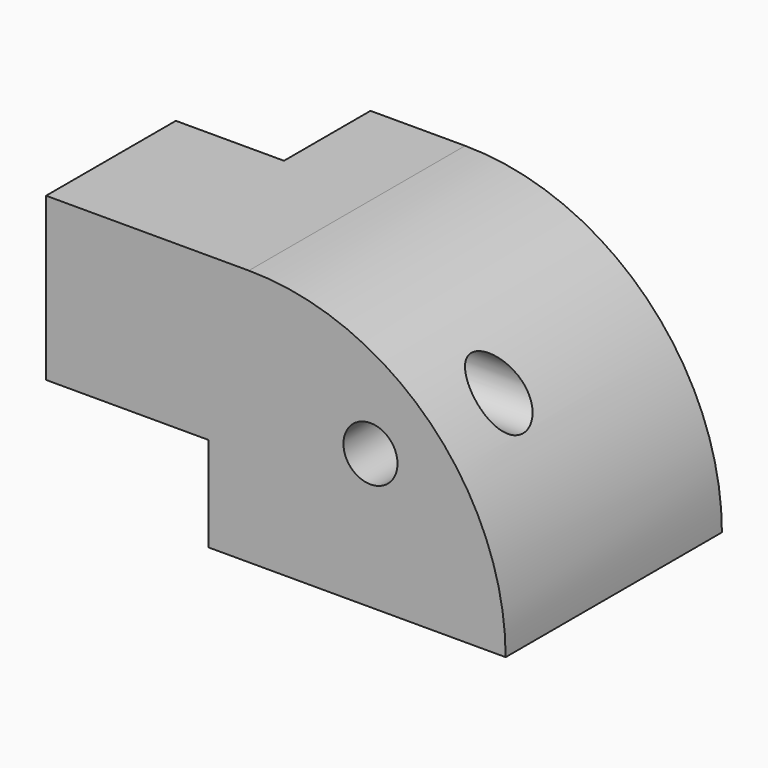
from build123d import *

# Parameters (mm, degrees)
F0_W      = 127
F0_H      = 120.65
F1_DEPTH  = 215.9
F2_W      = 76.2
F2_H      = 44.45
F3_DEPTH  = 127
F4_W      = 50.8
F4_H      = 76.2
F5_DEPTH  = 50.8
F8_D      = 25.4
F8_DEPTH  = 127
F8_TIP    = 7.6309298617
F9_R      = 120.64999
F10_DEPTH = 50.8
F13_D     = 25.4


# Not quite as in the source:
# - a fillet or chamfer is up to 0.001 mm smaller than in the source, because OpenCascade refuses the exact size
# - a feature of the source that left no trace in its solid (it failed there, or was rolled back) is left out


with BuildPart() as f1:
    # F0 (on Right) → F1 (new body)
    with BuildSketch(Plane.YZ):
        Rectangle(F0_W, F0_H)
    extrude(amount=F1_DEPTH)

    # F2 (on face) → F3 (cut)
    with BuildSketch(Plane.XZ.offset(63.5)):
        with Locations((38.1, -38.1)):
            Rectangle(F2_W, F2_H)
    extrude(amount=-F3_DEPTH, mode=Mode.SUBTRACT)

    # F4 (on face) → F5 (cut)
    with BuildSketch(Plane(origin=(0, 0, 0), x_dir=(0, -1, 0), z_dir=(-1, 0, 0))):
        with Locations((-38.1, 22.225)):
            Rectangle(F4_W, F4_H)
    extrude(amount=-F5_DEPTH, mode=Mode.SUBTRACT)

    # F8
    with Locations(Plane.XZ.offset(63.5)):
        with Locations((152.4, 3.175)):
            Hole(F8_D / 2, depth=F8_DEPTH)
            with Locations((0, 0, -(F8_DEPTH + F8_TIP / 2))):  # 118° drill point
                Cone(0, F8_D / 2, F8_TIP, mode=Mode.SUBTRACT)

    # F9 (radius 120.65 in the source; OpenCascade refuses exactly that, so slightly less here)
    f9_edges = [f1.edges().sort_by_distance(p)[0] for p in [
        (215.9, 0, 60.325),
    ]]
    fillet(f9_edges, radius=F9_R)

    # F4 (on face) → F10 (cut)
    with BuildSketch(Plane(origin=(0, 0, 0), x_dir=(0, -1, 0), z_dir=(-1, 0, 0))):
        with Locations((-38.1, 22.225)):
            Rectangle(F4_W, F4_H)
    extrude(amount=-F10_DEPTH, mode=Mode.SUBTRACT)

    # F13 (through all)
    with Locations(Plane(origin=(0, 0, 0), x_dir=(0, -1, 0), z_dir=(-1, 0, 0))):
        with Locations((25.4, 22.225)):
            Hole(F13_D / 2)


solid = f1.part
